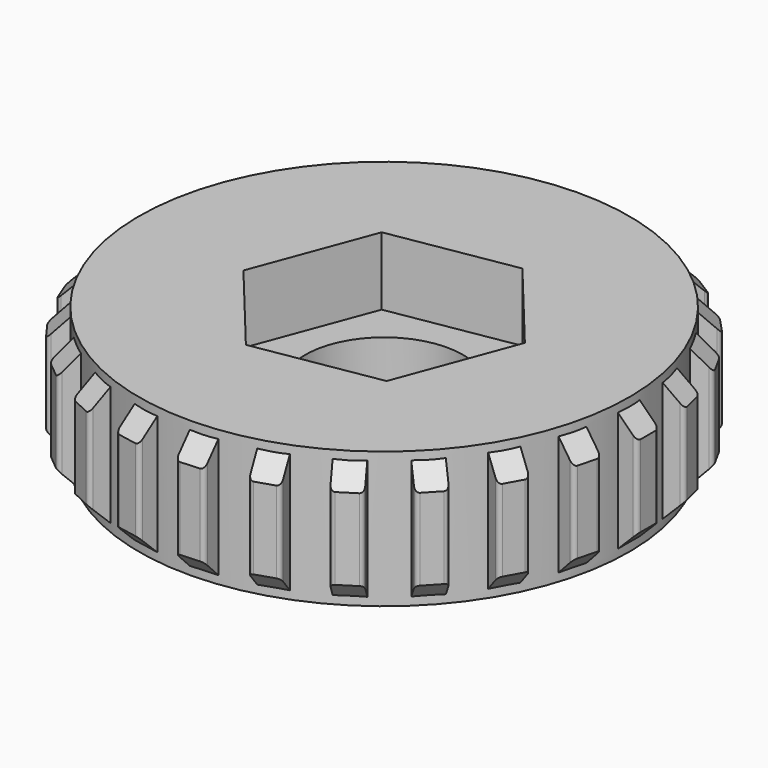
from build123d import *

# Parameters (mm, degrees)
F1_DEPTH    = 5
F2_R        = 0.15
F3_T1_DEPTH = 5.8433659759
F4_COUNT    = 25
F5_R        = 2.9
F6_DEPTH    = 5.001
F7_DEPTH    = 2.5


# Not quite as in the source:
# - a fillet or chamfer that OpenCascade refuses, or shapes differently, is made with other operations: its cross-section is extruded or revolved along the edge and cut away or added


with BuildPart() as f1:
    # F0 (on Top) → F1 (new body)
    with BuildSketch(Plane.XY):
        with BuildLine():
            ThreePointArc((8.9861003778, -0.5), (8.9965244234, -0.2500965811), (9, 0))
            ThreePointArc((9, 0), (8.9965244234, 0.2500965811), (8.9861003778, 0.5))
            ThreePointArc((8.9861003778, 0.5), (-9, 0), (8.9861003778, -0.5))
        make_face()
        with BuildLine():
            ThreePointArc((8.9861003778, 0.5), (8.9965244234, 0.2500965811), (9, 0))
            ThreePointArc((9, 0), (8.9965244234, -0.2500965811), (8.9861003778, -0.5))
            Line((8.9861003778, -0.5), (9.6871048306, -0.5))
            Line((9.6871048306, -0.5), (9.6871048306, 0.5))
            Line((9.6871048306, 0.5), (8.9861003778, 0.5))
        make_face()
    extrude(amount=F1_DEPTH)

    # F2
    f2_edges = [f1.edges().sort_by_distance(p)[0] for p in [
        (9.687105, -0.5, 2.5),
        (9.687105, 0.5, 2.5),
    ]]
    fillet(f2_edges, radius=F2_R)

    # F3: chamfer of 1 on 2 edges, made by hand

    # F3_s2 → F3_t1 (cut)
    with BuildSketch(Plane.XZ.offset(-2.921682988)):
        Polygon((8.6871048306, 0), (9.6871048306, 1), (9.6871048306, 0), align=None)
        Polygon((8.6871048306, 5), (9.6871048306, 4), (9.6871048306, 5), align=None)
    extrude(amount=F3_T1_DEPTH, mode=Mode.SUBTRACT)

    # F4: F1 ×25 about axis
    f4_axis = Axis((0, 0, 0), (0, 0, -1))


with BuildPart() as f1_1:
    add(f1.part)
    for i in range(1, F4_COUNT):
        add(f1.part.rotate(f4_axis, i * 360 / F4_COUNT))

    # F5 (on face) → F6 (cut, through all)
    with BuildSketch(Plane.XY.offset(5)):
        Circle(F5_R)
    extrude(amount=-F6_DEPTH, mode=Mode.SUBTRACT)

    # F5 (on face) → F7 (cut)
    with BuildSketch(Plane.XY.offset(5)):
        Polygon((2.9402983624, -3.5620189322), (4.5549480653, 0.7653636104), (1.6146497028, 4.3273825427), (-2.9402983624, 3.5620189322), (-4.5549480653, -0.7653636104), (-1.6146497028, -4.3273825427), align=None)
        Circle(F5_R, mode=Mode.SUBTRACT)
    extrude(amount=-F7_DEPTH, mode=Mode.SUBTRACT)


solid = f1_1.part
